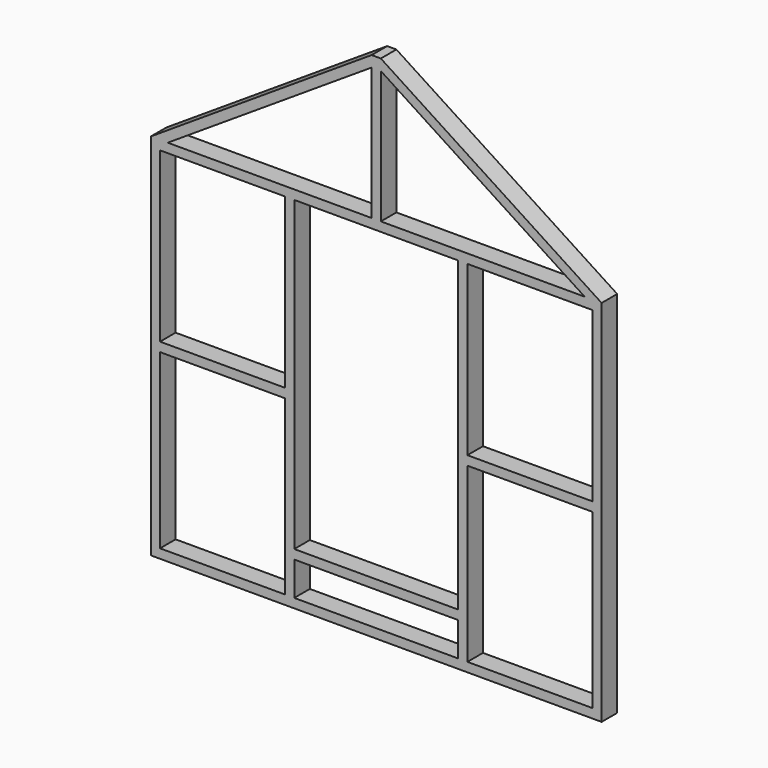
from build123d import *

# Parameters (mm, degrees)
F0_W     = 610
F0_H     = 45
F0_W_2   = 800
F1_DEPTH = 95


# Not quite as in the source:
# - a feature names something its author has since deleted; it is built from what else it names


with BuildPart() as f1:
    # F0 (on Front) → F1 (new body)
    with BuildSketch(Plane.XZ):
        Polygon((1100, -628.1681121112), (1100, -583.1681121112), (1055, -583.1681121112), (445, -583.1681121112), (400, -583.1681121112), (-400, -583.1681121112), (-445, -583.1681121112), (-1055, -583.1681121112), (-1100, -583.1681121112), (-1100, -628.1681121112), align=None)
        Polygon((1055, -583.1681121112), (1100, -583.1681121112), (1100, 1126.8318878888), (1055, 1126.8318878888), (1055, 304.8318878888), (1055, 259.8318878888), align=None)
        Polygon((1055, 1126.8318878888), (1100, 1126.8318878888), (1100, 1171.8318878888), (1017.398329114, 1171.8318878888), (22.5, 1171.8318878888), (-22.5, 1171.8318878888), (-1017.398329114, 1171.8318878888), (-1100, 1171.8318878888), (-1100, 1126.8318878888), (-1055, 1126.8318878888), (-445, 1126.8318878888), (-400, 1126.8318878888), (400, 1126.8318878888), (445, 1126.8318878888), align=None)
        Polygon((1017.398329114, 1171.8318878888), (1100, 1171.8318878888), (22.5, 1871.8318878888), (22.5, 1818.1695494942), align=None)
        Polygon((-1100, 1126.8318878888), (-1100, -583.1681121112), (-1055, -583.1681121112), (-1055, 259.8318878888), (-1055, 304.8318878888), (-1055, 1126.8318878888), align=None)
        Polygon((22.5, 1818.1695494942), (22.5, 1871.8318878888), (-22.5, 1871.8318878888), (-22.5, 1818.1695494942), (-22.5, 1171.8318878888), (22.5, 1171.8318878888), align=None)
        Polygon((-22.5, 1818.1695494942), (-22.5, 1871.8318878888), (-1100, 1171.8318878888), (-1017.398329114, 1171.8318878888), align=None)
        Polygon((-445, -583.1681121112), (-400, -583.1681121112), (-400, -418.1681121112), (-400, -373.1681121112), (-400, 1126.8318878888), (-445, 1126.8318878888), (-445, 304.8318878888), (-445, 259.8318878888), align=None)
        Polygon((400, -583.1681121112), (445, -583.1681121112), (445, 259.8318878888), (445, 304.8318878888), (445, 1126.8318878888), (400, 1126.8318878888), (400, -373.1681121112), (400, -418.1681121112), align=None)
        with Locations((750, 282.3318878888)):
            Rectangle(F0_W, F0_H)
        with Locations((-750, 282.3318878888)):
            Rectangle(F0_W, F0_H)
        with Locations((0, -395.6681121112)):
            Rectangle(F0_W_2, F0_H)
    extrude(amount=F1_DEPTH)


solid = f1.part
